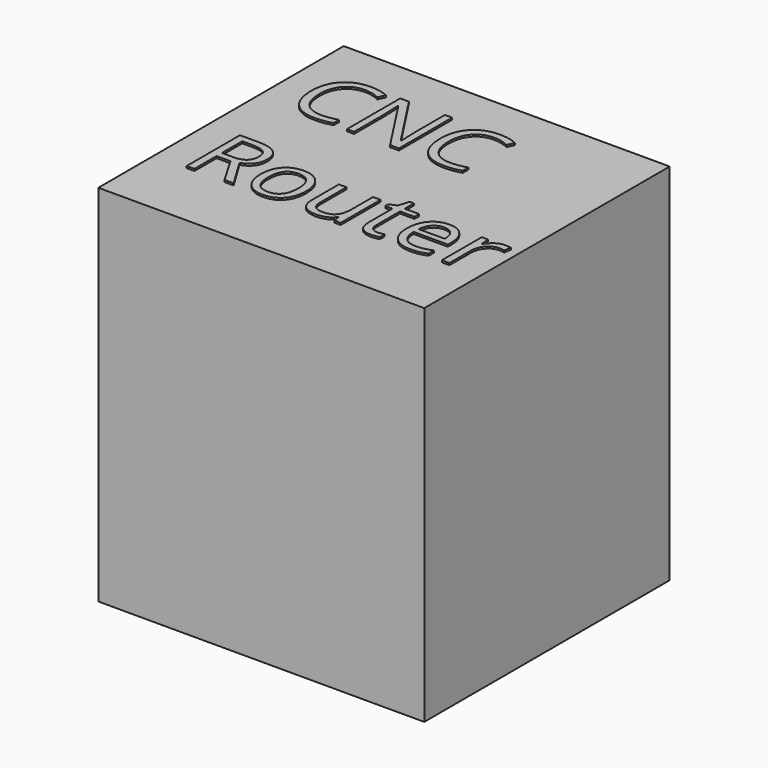
from build123d import *

# Parameters (mm, degrees)
F0_W         = 431.8
F0_H         = 406.4
F1_DEPTH     = 482.6
F2_TEXT_SIZE = 123.4722222222
F3_DEPTH     = 2.54


# Not quite as in the source:
# - Text() gives the source's letters only with a copy of the font that has no kerning and outlines rounded to 1/6400 em; it was checked with that copy


with BuildPart() as f1:
    # F0 (on Top) → F1 (new body)
    with BuildSketch(Plane.XY):
        with Locations((6.242138142, 0)):
            Rectangle(F0_W, F0_H)
    extrude(amount=F1_DEPTH)

    # F2 (on face) → F3 (join)
    with BuildSketch(Plane.XY.offset(482.6)):
        with Locations((-177.7973398007, 56.152101936)):
            Text('CNC', F2_TEXT_SIZE, font='Open Sans', text_align=(TextAlign.LEFT, TextAlign.BOTTOM))
        with Locations((-177.7973398007, -111.7701202862)):
            Text('Router', F2_TEXT_SIZE, font='Open Sans', text_align=(TextAlign.LEFT, TextAlign.BOTTOM))
    extrude(amount=F3_DEPTH)


solid = f1.part
